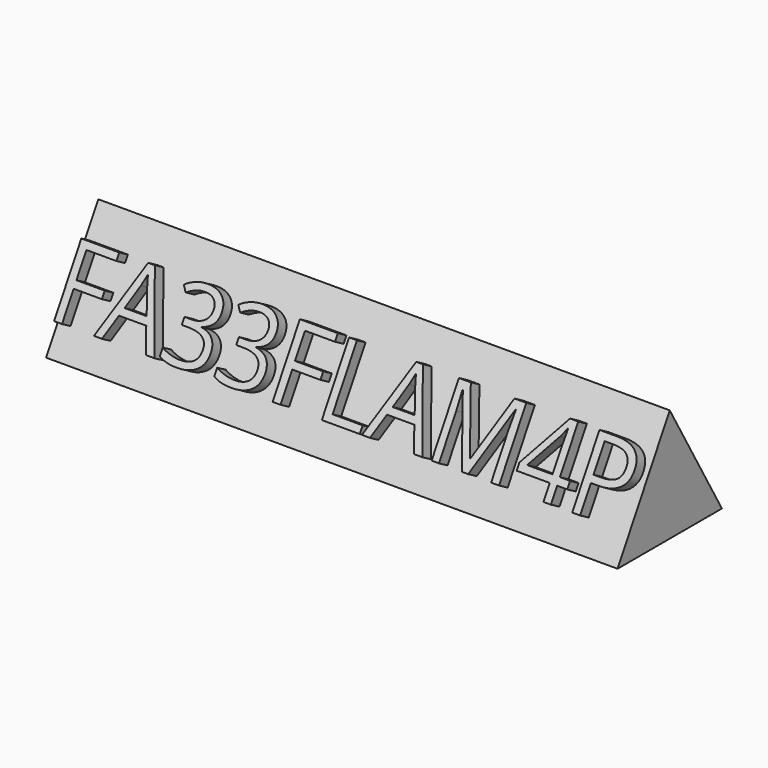
from build123d import *

# Parameters (mm, degrees)
F1_DEPTH     = 46
F2_TEXT_SIZE = 7.6739421477
F3_DEPTH     = 1


# Not quite as in the source:
# - Text() gives the source's letters only with a copy of the font that has no kerning and outlines rounded to 1/6400 em; it was checked with that copy


with BuildPart() as f1:
    # F0 (on Right) → F1 (new body)
    with BuildSketch(Plane.YZ):
        Polygon((0, 6.0621778265), (-5.25, -3.0310889132), (5.25, -3.0310889132), align=None)
    extrude(amount=F1_DEPTH)

    # F2 (on face) → F3 (join)
    with BuildSketch(Plane(origin=(0, -2.625, 1.5155444566), x_dir=(1, 0, 0), z_dir=(0, -0.8660254038, 0.5))):
        with Locations((-0.3741590772, -2.8536943719)):
            Text('FA33FLAM4P', F2_TEXT_SIZE, font='Open Sans', text_align=(TextAlign.LEFT, TextAlign.BOTTOM))
    extrude(amount=F3_DEPTH)


solid = f1.part
